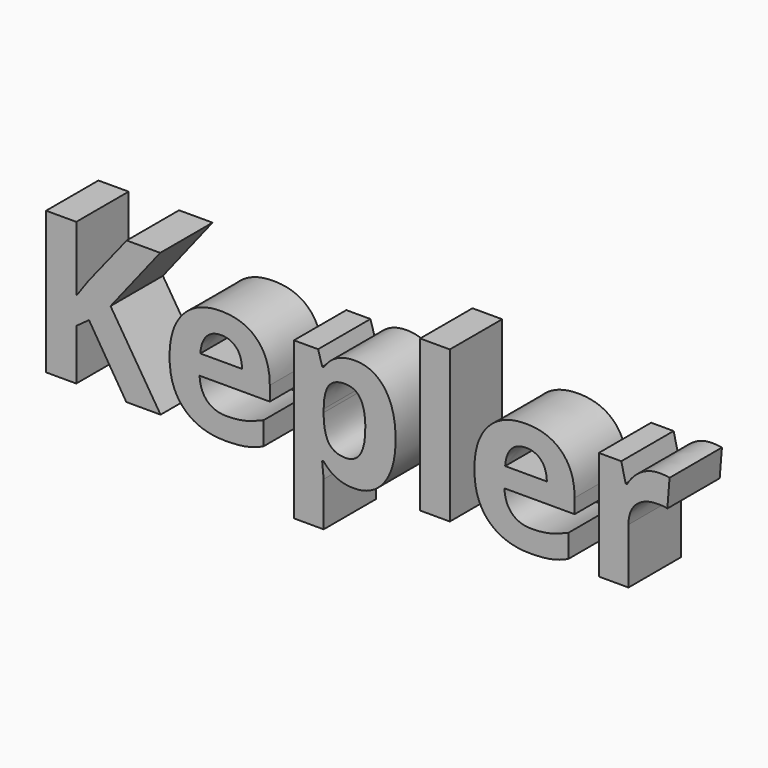
from build123d import *

# Parameters (mm, degrees)
F0_TEXT_SIZE = 9.1419864775
F1_DEPTH     = 3


# Not quite as in the source:
# - Text() gives the source's letters only with a copy of the font that has no kerning and outlines rounded to 1/6400 em; it was checked with that copy


with BuildPart() as f1:
    # F0 (on Front) → F1 (new body)
    with BuildSketch(Plane.XZ):
        with Locations((-5.5948959529, -2.6855498859)):
            Text('Kepler', F0_TEXT_SIZE, font='Open Sans', font_style=FontStyle.BOLD, text_align=(TextAlign.LEFT, TextAlign.BOTTOM))
    extrude(amount=F1_DEPTH)


solid = f1.part
